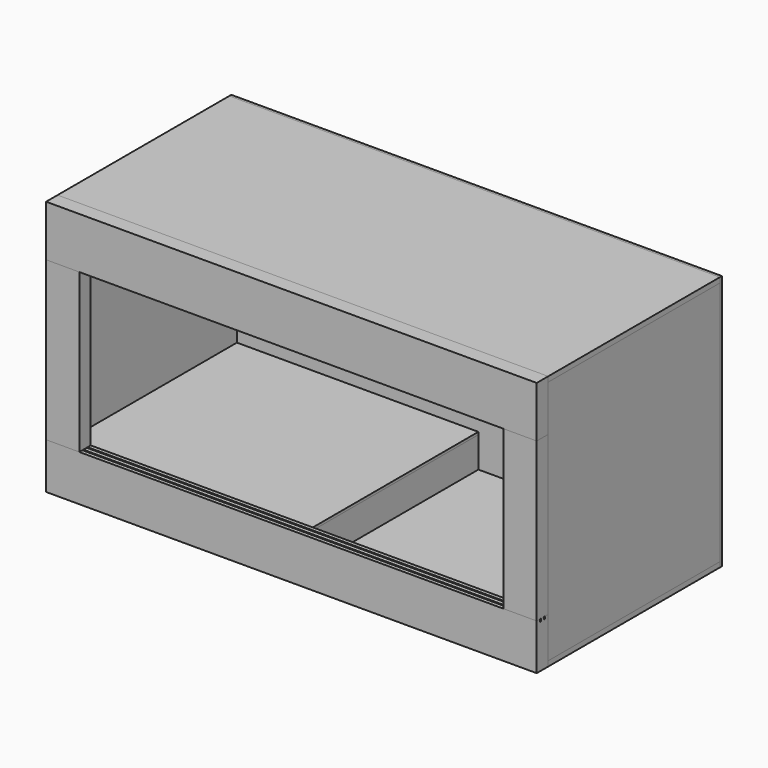
from build123d import *

# Parameters (mm, degrees)
F0_W      = 1219.2
F0_H      = 533.4
F1_DEPTH  = 19.05
F2_W      = 19.05
F2_H      = 533.4
F3_DEPTH  = 6.35
F4_W      = 19.05
F4_H      = 533.4
F5_DEPTH  = 609.6
F6_R      = 9.525
F7_DEPTH  = 12.7
F9_W      = 19.05
F9_H      = 533.4
F9_W_2    = 1200.15
F10_DEPTH = 12.7
F11_W     = 1181.1
F11_H     = 533.4
F12_DEPTH = 6.35
F14_DEPTH = 6.35
F16_DEPTH = 35.56
F18_DEPTH = 35.56
F19_W     = 63.5
F19_H     = 393.7
F19_W_2   = 19.05
F20_DEPTH = 35.56
F22_W     = 19.05
F22_H     = 533.4
F23_DEPTH = 76.2
F25_W     = 581.025
F25_H     = 533.4
F25_W_2   = 19.05
F26_DEPTH = 6.35
F27_W     = 1219.2
F27_H     = 3.175
F28_DEPTH = 6.35


with BuildPart() as f1:
    # F0 (on Top) → F1 (new body)
    with BuildSketch(Plane.XY):
        Rectangle(F0_W, F0_H)
    extrude(amount=F1_DEPTH)

    # F2 (on face) → F3 (cut)
    with BuildSketch(Plane.XY.offset(19.05)):
        with Locations((-600.075, 0)):
            Rectangle(F2_W, F2_H)
        with Locations((600.075, 0)):
            Rectangle(F2_W, F2_H)
    extrude(amount=-F3_DEPTH, mode=Mode.SUBTRACT)


with BuildPart() as f5:
    # F4 (on face) → F5 (new body)
    with BuildSketch(Plane.XY.offset(12.7)):
        with Locations((-600.075, 0)):
            Rectangle(F4_W, F4_H)
    extrude(amount=F5_DEPTH)

    # F6 (on face) → F7 (cut)
    with BuildSketch(Plane.YZ.offset(-590.55)):
        with Locations((-237.3699372192, 571.5)):
            Circle(F6_R)
        with Locations((-236.7096560535, 444.5)):
            Circle(F6_R)
        with Locations((-233.8235423241, 203.2)):
            Circle(F6_R)
        with Locations((-235.7480174049, 76.2)):
            Circle(F6_R)
        with Locations((-238.5504677733, 323.85)):
            Circle(F6_R)
    extrude(amount=-F7_DEPTH, mode=Mode.SUBTRACT)


with BuildPart() as f8_1:
    # F8: instance of F5
    add(f5.part.mirror(Plane.YZ))


with BuildPart() as f10:
    # F9 (on face) → F10 (new body)
    with BuildSketch(Plane.XY.offset(622.3)):
        with Locations((-600.075, 0)):
            Rectangle(F9_W, F9_H)
        with Locations((9.525, 0)):
            Rectangle(F9_W_2, F9_H)
    extrude(amount=F10_DEPTH)

    # F11 (on face) → F12 (join)
    with BuildSketch(Plane(origin=(0, 0, 622.3), x_dir=(1, 0, 0), z_dir=(0, 0, -1))):
        Rectangle(F11_W, F11_H)
    extrude(amount=F12_DEPTH)


with BuildPart() as f14:
    # F13 (on face) → F14 (new body)
    with BuildSketch(Plane(origin=(0, 266.7, 0), x_dir=(-1, 0, 0), z_dir=(0, 1, 0))):
        Polygon((-590.55, 622.3), (-609.6, 622.3), (-609.6, 0), (609.6, 0), (609.6, 622.3), (590.55, 622.3), (590.55, 615.95), (-590.55, 615.95), align=None)
        Polygon((609.6, 635), (-609.6, 635), (-609.6, 622.3), (-590.55, 622.3), (-590.55, 615.95), (590.55, 615.95), (590.55, 622.3), (609.6, 622.3), align=None)
    extrude(amount=F14_DEPTH)


with BuildPart() as f16:
    # F15 (on face) → F16 (new body)
    with BuildSketch(Plane.XZ.offset(266.7)):
        Polygon((-609.6, 114.3), (-609.6, 12.7), (-590.55, 12.7), (-590.55, 19.05), (590.55, 19.05), (590.55, 12.7), (609.6, 12.7), (609.6, 114.3), align=None)
        Polygon((-609.6, 12.7), (-609.6, 0), (609.6, 0), (609.6, 12.7), (590.55, 12.7), (590.55, 19.05), (-590.55, 19.05), (-590.55, 12.7), align=None)
    extrude(amount=F16_DEPTH)

    # F27 (on face) → F28 (cut)
    with BuildSketch(Plane.XY.offset(114.3)):
        with Locations((0, -277.8125)):
            Rectangle(F27_W, F27_H)
        with Locations((0, -291.1475)):
            Rectangle(F27_W, F27_H)
    extrude(amount=-F28_DEPTH, mode=Mode.SUBTRACT)


with BuildPart() as f18:
    # F17 (on face) → F18 (new body)
    with BuildSketch(Plane.XZ.offset(266.7)):
        Polygon((609.6, 508), (609.6, 622.3), (590.55, 622.3), (590.55, 615.95), (-590.55, 615.95), (-590.55, 622.3), (-609.6, 622.3), (-609.6, 508), align=None)
        Polygon((609.6, 622.3), (609.6, 635), (-609.6, 635), (-609.6, 622.3), (-590.55, 622.3), (-590.55, 615.95), (590.55, 615.95), (590.55, 622.3), align=None)
    extrude(amount=F18_DEPTH)


with BuildPart() as f20:
    # F19 (on face) → F20 (new body)
    with BuildSketch(Plane.XZ.offset(266.7)):
        with Locations((-558.8, 311.15)):
            Rectangle(F19_W, F19_H)
        with Locations((-600.075, 311.15)):
            Rectangle(F19_W_2, F19_H)
    extrude(amount=F20_DEPTH)


with BuildPart() as f21_1:
    # F21: instance of F20
    add(f20.part.mirror(Plane.YZ))


with BuildPart() as f23:
    # F22 (on face) → F23 (new body)
    with BuildSketch(Plane.XY.offset(19.05)):
        Rectangle(F22_W, F22_H)
    extrude(amount=F23_DEPTH)


with BuildPart() as f24_1:
    # F24: copy of F23
    add(f23.part.moved(Location((-558.8, 0, 0))))


with BuildPart() as f26:
    # F25 (on face) → F26 (new body)
    with BuildSketch(Plane.XY.offset(95.25)):
        with Locations((-300.0375, 0)):
            Rectangle(F25_W, F25_H)
        Rectangle(F25_W_2, F25_H)
    extrude(amount=F26_DEPTH)


solid = Compound([f1.part, f5.part, f8_1.part, f10.part, f14.part, f16.part, f18.part, f20.part, f21_1.part, f23.part, f24_1.part, f26.part])
